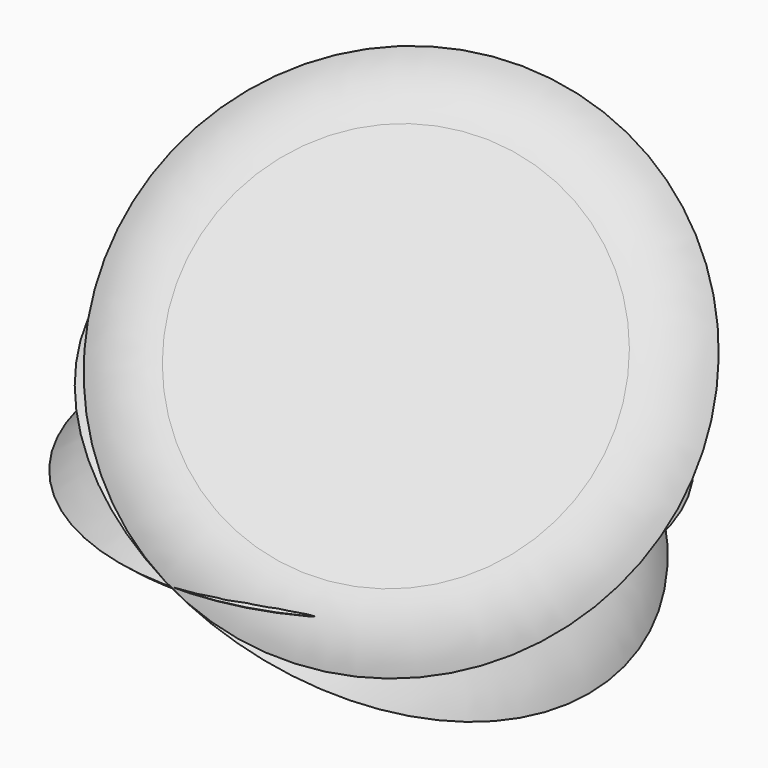
from build123d import *

# Parameters (mm, degrees)
F0_R      = 12.7
F1_DEPTH  = 1.27
F2_SIZE   = 1.26999
F8_ANGLE  = -30
F11_ANGLE = -45


# Not quite as in the source:
# - a fillet or chamfer that OpenCascade refuses, or shapes differently, is made with other operations: its cross-section is extruded or revolved along the edge and cut away or added
# - a fillet or chamfer is up to 0.001 mm smaller than in the source, because OpenCascade refuses the exact size


with BuildPart() as f1:
    # F0 (on Top) → F1 (new body, symmetric)
    with BuildSketch(Plane.XY):
        Circle(F0_R)
    extrude(amount=F1_DEPTH, both=True)

    # F2 (size 1.27 in the source; OpenCascade refuses exactly that, so slightly less here)
    f2_edges = [f1.edges().sort_by_distance(p)[0] for p in [
        (-12.7, 0, -1.27),
        (-12.7, 0, 1.27),
    ]]
    chamfer(f2_edges, length=F2_SIZE)

    # F3: fillet of radius 5.08 on 1 edges, made by hand

    # F3_s1 → F3_t2 (revolve, cut)
    with BuildSketch(Plane.XZ):
        with BuildLine():
            ThreePointArc((12.7, 1e-05), (11.135951327, 0.9419075538), (9.3399071739, 1.27))
            Line((9.3399071739, 1.27), (11.43001, 1.27))
            Line((11.43001, 1.27), (12.7, 1e-05))
        make_face()
    revolve(axis=Axis((0, 0, 1.27), (0, 0, 1)), mode=Mode.SUBTRACT)

    # F4: fillet of radius 5.08 on 1 edges, made by hand

    # F4_s1 → F4_t2 (revolve, cut)
    with BuildSketch(Plane.XZ):
        with BuildLine():
            ThreePointArc((12.7, -1e-05), (11.135951327, -0.9419075538), (9.3399071739, -1.27))
            Line((9.3399071739, -1.27), (11.43001, -1.27))
            Line((11.43001, -1.27), (12.7, -1e-05))
        make_face()
    revolve(axis=Axis((0, 0, -1.27), (0, 0, 1)), mode=Mode.SUBTRACT)


with BuildPart() as f5_1:
    # F5: copy of F1
    add(f1.part)


with BuildPart() as f5_1_1:
    # F8: moved
    add(f5_1.part.rotate(Axis((0, 17.4700720236, 0), (0, -1, 0)), F8_ANGLE))


with BuildPart() as f11_1:
    # F11: copy of F5_1
    add(f5_1_1.part.rotate(Axis((34.8542153159, -12.7, -20.123090595), (-0.8660254038, 0, 0.5)), F11_ANGLE))


solid = Compound([f1.part, f5_1_1.part, f11_1.part])
